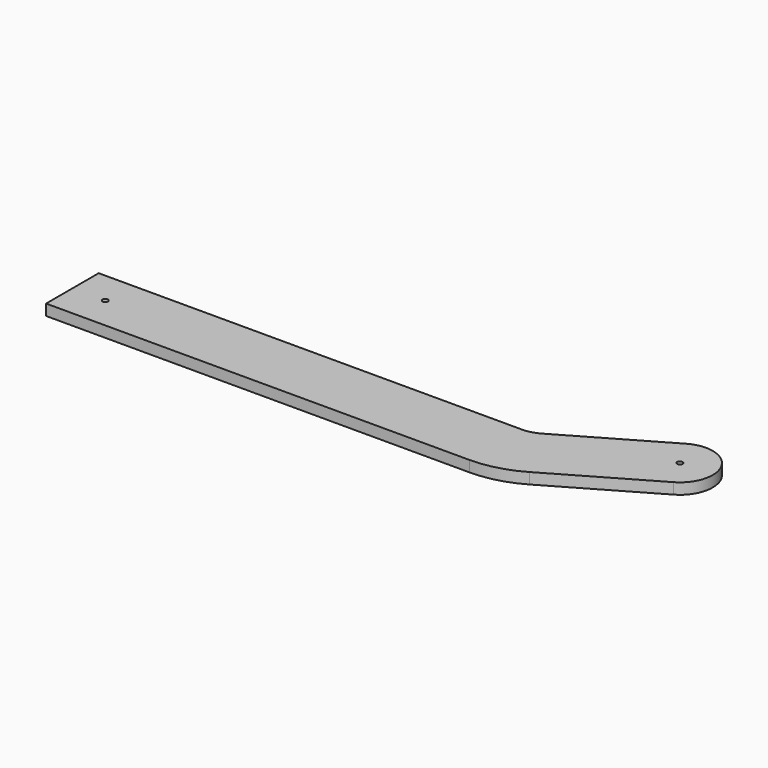
from build123d import *

# Parameters (mm, degrees)
F0_R     = 3.175
F1_DEPTH = 6.35


# Not quite as in the source:
# - a feature names something its author has since deleted; it is built from what else it names


with BuildPart() as f1:
    # F0 (on Top) → F1 (new body, symmetric)
    with BuildSketch(Plane.XY):
        with BuildLine():
            Line((245.237, 38.1), (-245.237, 38.1))
            Line((-245.237, 38.1), (-245.237, -38.1))
            Line((-245.237, -38.1), (245.237, -38.1))
            ThreePointArc((245.237, -38.1), (274.8200168552, -34.2053219448), (302.387, -22.7867036526))
            Line((302.387, -22.7867036526), (416.687, 43.2044321158))
            ThreePointArc((416.687, 43.2044321158), (430.6325678842, 95.25), (378.587, 109.1955678842))
            Line((378.587, 109.1955678842), (321.437, 76.2))
            Line((321.437, 76.2), (264.287, 43.2044321158))
            ThreePointArc((264.287, 43.2044321158), (255.0980056184, 39.3982260184), (245.237, 38.1))
        make_face()
        with Locations((-207.137, 0)):
            Circle(F0_R, mode=Mode.SUBTRACT)
        with BuildLine():
            ThreePointArc((394.887369343, 74.6125), (396.8152495318, 79.2668144985), (400.812, 76.2))
            ThreePointArc((400.812, 76.2), (398.4587504682, 73.1331855015), (394.887369343, 74.6125))
        make_face(mode=Mode.SUBTRACT)
    extrude(amount=F1_DEPTH, both=True)


solid = f1.part
